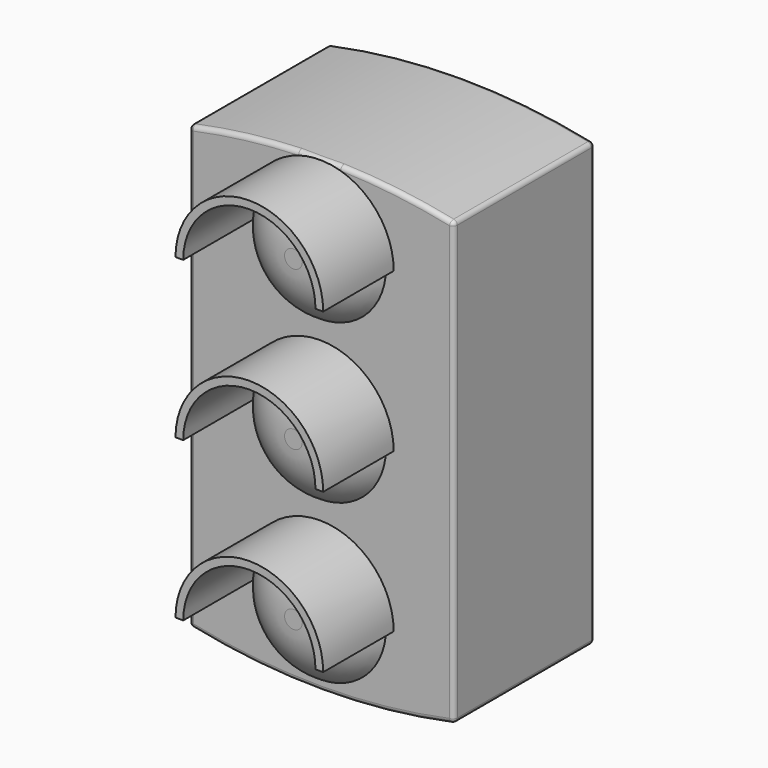
from build123d import *

# Parameters (mm, degrees)
F0_R     = 19.05
F1_DEPTH = 50.8
F2_DEPTH = 58.42
F5_DEPTH = 25.4
F6_R     = 1.27
F8_DEPTH = 9.525


# Not quite as in the source:
# - a fillet or chamfer that OpenCascade refuses, or shapes differently, is made with other operations: its cross-section is extruded or revolved along the edge and cut away or added


with BuildPart() as f1:
    # F0 (on Front) → F1 (new body)
    with BuildSketch(Plane.XZ):
        with BuildLine():
            ThreePointArc((26.4360774308, 56.4342959829), (-11.7042224138, 60.4920635507), (-49.8445222585, 56.4342959829))
            Line((-49.8445222585, 56.4342959829), (-49.8445222585, -70.5657040171))
            ThreePointArc((-49.8445222585, -70.5657040171), (-11.7042224138, -74.6371140825), (26.4360774308, -70.5657040171))
            Line((26.4360774308, -70.5657040171), (26.4360774308, 56.4342959829))
        make_face()
        with Locations((-12.1294902638, -52.7166463435)):
            Circle(F0_R, mode=Mode.SUBTRACT)
        with Locations((-12.1294902638, -6.9966463435)):
            Circle(F0_R, mode=Mode.SUBTRACT)
        with Locations((-12.1294902638, 38.7233536565)):
            Circle(F0_R, mode=Mode.SUBTRACT)
    extrude(amount=F1_DEPTH)

    # F0 (on Front) → F2 (join)
    with BuildSketch(Plane.XZ):
        with Locations((-12.1294902638, 38.7233536565)):
            Circle(F0_R)
        with Locations((-12.1294902638, -6.9966463435)):
            Circle(F0_R)
        with Locations((-12.1294902638, -52.7166463435)):
            Circle(F0_R)
    extrude(amount=F2_DEPTH)

    # F3: fillet of radius 27.5971 on 3 edges, made by hand

    # F3_s1 → F3_t2 (revolve, cut)
    with BuildSketch(Plane.XY.offset(38.7233536565)):
        with BuildLine():
            ThreePointArc((6.9205097362, -50.8), (-1.8653063418, -56.4442773519), (-12.119327553, -58.42))
            Line((-12.119327553, -58.42), (6.9205097362, -58.42))
            Line((6.9205097362, -58.42), (6.9205097362, -50.8))
        make_face()
    revolve(axis=Axis((-12.1294902638, -58.42, 38.7233536565), (0, -1, 0)), mode=Mode.SUBTRACT)

    # F3_s3 → F3_t4 (revolve, cut)
    with BuildSketch(Plane.XY.offset(-6.9966463435)):
        with BuildLine():
            ThreePointArc((6.9205097362, -50.8), (-1.8653063418, -56.4442773519), (-12.119327553, -58.42))
            Line((-12.119327553, -58.42), (6.9205097362, -58.42))
            Line((6.9205097362, -58.42), (6.9205097362, -50.8))
        make_face()
    revolve(axis=Axis((-12.1294902638, -58.42, -6.9966463435), (0, -1, 0)), mode=Mode.SUBTRACT)

    # F3_s5 → F3_t6 (revolve, cut)
    with BuildSketch(Plane.XY.offset(-52.7166463435)):
        with BuildLine():
            ThreePointArc((6.9205097362, -50.8), (-1.8653063418, -56.4442773519), (-12.119327553, -58.42))
            Line((-12.119327553, -58.42), (6.9205097362, -58.42))
            Line((6.9205097362, -58.42), (6.9205097362, -50.8))
        make_face()
    revolve(axis=Axis((-12.1294902638, -58.42, -52.7166463435), (0, -1, 0)), mode=Mode.SUBTRACT)

    # F4 (on face) → F5 (join)
    with BuildSketch(Plane.XZ.offset(50.8)):
        with BuildLine():
            ThreePointArc((-31.1794902638, 38.7233536565), (-12.1294902638, 57.7733536565), (6.9205097362, 38.7233536565))
            Line((6.9205097362, 38.7233536565), (9.1469490083, 38.7233536565))
            ThreePointArc((9.1469490083, 38.7233536565), (-12.1294902638, 59.9997929286), (-33.4059295358, 38.7233536565))
            Line((-33.4059295358, 38.7233536565), (-31.1794902638, 38.7233536565))
        make_face()
        with BuildLine():
            Line((6.9205097362, -6.9966463435), (9.1430097362, -6.9966463435))
            ThreePointArc((9.1430097362, -6.9966463435), (-12.1294902638, 14.2758536565), (-33.4019902638, -6.9966463435))
            Line((-33.4019902638, -6.9966463435), (-31.1794902638, -6.9966463435))
            ThreePointArc((-31.1794902638, -6.9966463435), (-12.1294902638, 12.0533536565), (6.9205097362, -6.9966463435))
        make_face()
        with BuildLine():
            Line((6.9205097362, -52.7166463435), (9.1430097362, -52.7166463435))
            ThreePointArc((9.1430097362, -52.7166463435), (-12.1294902638, -31.4441463435), (-33.4019902638, -52.7166463435))
            Line((-33.4019902638, -52.7166463435), (-31.1794902638, -52.7166463435))
            ThreePointArc((-31.1794902638, -52.7166463435), (-12.1294902638, -33.6666463435), (6.9205097362, -52.7166463435))
        make_face()
    extrude(amount=F5_DEPTH)

    # F6
    f6_edges = [f1.edges().sort_by_distance(p)[0] for p in [
        (26.436077, -50.8, -7.065704),
        (-11.704222, -50.8, -74.637114),
        (26.436077, -25.4, -70.565704),
        (-49.844522, -25.4, -70.565704),
        (-11.704222, 0, -74.637114),
        (26.436077, 0, -7.065704),
        (-49.844522, -50.8, -7.065704),
        (-49.844522, 0, -7.065704),
        (-11.704222, -50.8, 60.492064),
        (-11.704222, 0, 60.492064),
        (-49.844522, -25.4, 56.434296),
        (26.436077, -25.4, 56.434296),
    ]]
    fillet(f6_edges, radius=F6_R)


with BuildPart() as f8:
    # F7 (on face) → F8 (new body)
    with BuildSketch(Plane.XZ.offset(50.8)):
        with BuildLine():
            ThreePointArc((6.9205097362, 38.7233536565), (-12.1294902638, 57.7733536565), (-31.1794902638, 38.7233536565))
            ThreePointArc((-31.1794902638, 38.7233536565), (-12.1294902638, 19.6733536565), (6.9205097362, 38.7233536565))
        make_face()
    extrude(amount=F8_DEPTH)

    # F9: fillet of radius 19.05 on 1 edges, made by hand

    # F9_s1 → F9_t2 (revolve, cut)
    with BuildSketch(Plane.XY.offset(38.7233536565)):
        with BuildLine():
            ThreePointArc((6.9205097362, -50.8), (-0.0522742059, -57.7727839421), (-9.5772742059, -60.325))
            Line((-9.5772742059, -60.325), (6.9205097362, -60.325))
            Line((6.9205097362, -60.325), (6.9205097362, -50.8))
        make_face()
    revolve(axis=Axis((-12.1294902638, -60.325, 38.7233536565), (0, 1, 0)), mode=Mode.SUBTRACT)


with BuildPart() as f8b:
    # F7 (on face) → F8, piece 2 (new body)
    with BuildSketch(Plane.XZ.offset(50.8)):
        with BuildLine():
            ThreePointArc((-31.1794902638, -6.9966463435), (-12.1294902638, -26.0466463435), (6.9205097362, -6.9966463435))
            ThreePointArc((6.9205097362, -6.9966463435), (-12.1294902638, 12.0533536565), (-31.1794902638, -6.9966463435))
        make_face()
    extrude(amount=F8_DEPTH)

    # F9#2: fillet of radius 19.05 on 1 edges, made by hand

    # F9_2_s1 → F9_2_t2 (revolve, cut)
    with BuildSketch(Plane.XY.offset(-6.9966463435)):
        with BuildLine():
            ThreePointArc((6.9205097362, -50.8), (-0.0522742059, -57.7727839421), (-9.5772742059, -60.325))
            Line((-9.5772742059, -60.325), (6.9205097362, -60.325))
            Line((6.9205097362, -60.325), (6.9205097362, -50.8))
        make_face()
    revolve(axis=Axis((-12.1294902638, -60.325, -6.9966463435), (0, 1, 0)), mode=Mode.SUBTRACT)


with BuildPart() as f8c:
    # F7 (on face) → F8, piece 3 (new body)
    with BuildSketch(Plane.XZ.offset(50.8)):
        with BuildLine():
            ThreePointArc((-31.1794902638, -52.7166463435), (-12.1294902638, -71.7666463435), (6.9205097362, -52.7166463435))
            ThreePointArc((6.9205097362, -52.7166463435), (-12.1294902638, -33.6666463435), (-31.1794902638, -52.7166463435))
        make_face()
    extrude(amount=F8_DEPTH)

    # F9#3: fillet of radius 19.05 on 1 edges, made by hand

    # F9_3_s1 → F9_3_t2 (revolve, cut)
    with BuildSketch(Plane.XY.offset(-52.7166463435)):
        with BuildLine():
            ThreePointArc((-31.1794902638, -50.8), (-24.2067063217, -57.7727839421), (-14.6817063217, -60.325))
            Line((-14.6817063217, -60.325), (-31.1794902638, -60.325))
            Line((-31.1794902638, -60.325), (-31.1794902638, -50.8))
        make_face()
    revolve(axis=Axis((-12.1294902638, -60.325, -52.7166463435), (0, 1, 0)), mode=Mode.SUBTRACT)


solid = Compound([f1.part, f8.part, f8b.part, f8c.part])
